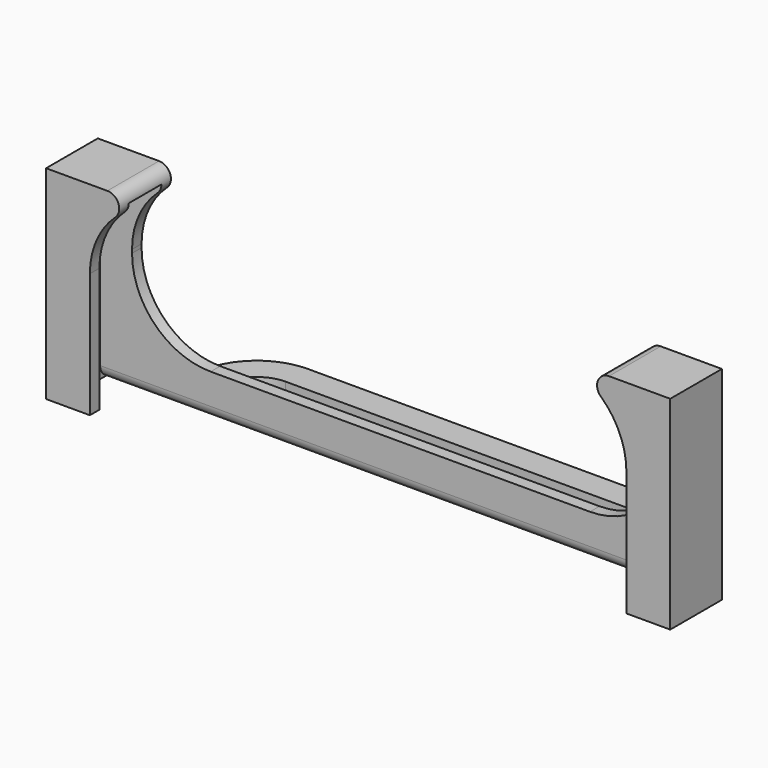
from build123d import *

# Parameters (mm, degrees)
F4_DEPTH     = 2.8
F5_W         = 146.8
F5_H         = 15.2
F5_W_2       = 141.2
F5_H_2       = 9.6
F6_DEPTH     = 47.8
F8_DEPTH     = 15.201
F9_DEPTH     = 2.8
F10_DEPTH    = 15.2
F11_T1_DEPTH = 141.2
F11_T3_DEPTH = 87.1722168618


# Not quite as in the source:
# - a fillet or chamfer that OpenCascade refuses, or shapes differently, is made with other operations: its cross-section is extruded or revolved along the edge and cut away or added
# - a feature names something its author has since deleted; it is built from what else it names


with BuildPart() as f4:
    # F3 (on Top) → F4 (new body)
    with BuildSketch(Plane.XY):
        with BuildLine():
            ThreePointArc((55, 5), (50.6066017178, 15.6066017178), (40, 20))
            Line((40, 20), (-40, 20))
            ThreePointArc((-40, 20), (-50.6066017178, 15.6066017178), (-55, 5))
            Line((-55, 5), (-55, 0))
            Line((-55, 0), (55, 0))
            Line((55, 0), (55, 5))
        make_face()
        with BuildLine():
            ThreePointArc((-48.3666002653, 6.5), (-45.4543560573, 11.5192024052), (-40, 13.5))
            Line((-40, 13.5), (40, 13.5))
            ThreePointArc((40, 13.5), (45.4543560573, 11.5192024052), (48.3666002653, 6.5))
            Line((48.3666002653, 6.5), (-48.3666002653, 6.5))
        make_face(mode=Mode.SUBTRACT)
    extrude(amount=F4_DEPTH)

    # F5 (on Top) → F6 (join)
    with BuildSketch(Plane.XY):
        with Locations((0, -7.6)):
            Rectangle(F5_W, F5_H)
        with Locations((0, -7.6)):
            Rectangle(F5_W_2, F5_H_2, mode=Mode.SUBTRACT)
    extrude(amount=F6_DEPTH)

    # F7 (on Front) → F8 (cut, through all)
    with BuildSketch(Plane.XZ):
        with BuildLine():
            Line((44.6, 47.8), (-44.6, 47.8))
            ThreePointArc((-44.6, 47.8), (-49.68920426, 47.0862306293), (-54.3857038582, 45))
            Line((-54.3857038582, 45), (54.3857038582, 45))
            ThreePointArc((54.3857038582, 45), (49.68920426, 47.0862306293), (44.6, 47.8))
        make_face()
        with BuildLine():
            ThreePointArc((-44.6, 10), (-57.681475452, 15.418524548), (-63.1, 28.5))
            Line((-63.1, 28.5), (-63.1, 10))
            Line((-63.1, 10), (-63.1, 0))
            Line((-63.1, 0), (63.1, 0))
            Line((63.1, 0), (63.1, 10))
            Line((63.1, 10), (63.1, 28.5))
            ThreePointArc((63.1, 28.5), (57.681475452, 15.418524548), (44.6, 10))
            Line((44.6, 10), (-44.6, 10))
        make_face()
        with BuildLine():
            Line((54.3857038582, 45), (-54.3857038582, 45))
            ThreePointArc((-54.3857038582, 45), (-60.7753751328, 38.2781534467), (-63.1, 29.3))
            Line((-63.1, 29.3), (-63.1, 28.5))
            ThreePointArc((-63.1, 28.5), (-57.681475452, 15.418524548), (-44.6, 10))
            Line((-44.6, 10), (44.6, 10))
            ThreePointArc((44.6, 10), (57.681475452, 15.418524548), (63.1, 28.5))
            Line((63.1, 28.5), (63.1, 29.3))
            ThreePointArc((63.1, 29.3), (60.7753751328, 38.2781534467), (54.3857038582, 45))
        make_face()
    extrude(amount=F8_DEPTH, mode=Mode.SUBTRACT)

    # F7 (on Front) → F9 (join)
    with BuildSketch(Plane.XZ):
        with BuildLine():
            ThreePointArc((-44.6, 10), (-57.681475452, 15.418524548), (-63.1, 28.5))
            Line((-63.1, 28.5), (-63.1, 10))
            Line((-63.1, 10), (-63.1, 0))
            Line((-63.1, 0), (63.1, 0))
            Line((63.1, 0), (63.1, 10))
            Line((63.1, 10), (63.1, 28.5))
            ThreePointArc((63.1, 28.5), (57.681475452, 15.418524548), (44.6, 10))
            Line((44.6, 10), (-44.6, 10))
        make_face()
    extrude(amount=F9_DEPTH)

    # F7 (on Front) → F10 (join)
    with BuildSketch(Plane.XZ):
        with BuildLine():
            ThreePointArc((-54.3857038582, 45), (-49.68920426, 47.0862306293), (-44.6, 47.8))
            Line((-44.6, 47.8), (-63.1, 47.8))
            Line((-63.1, 47.8), (-73.4, 47.8))
            Line((-73.4, 47.8), (-73.4, 45))
            Line((-73.4, 45), (-54.3857038582, 45))
        make_face()
        with BuildLine():
            Line((63.1, 47.8), (44.6, 47.8))
            ThreePointArc((44.6, 47.8), (49.68920426, 47.0862306293), (54.3857038582, 45))
            Line((54.3857038582, 45), (73.4, 45))
            Line((73.4, 45), (73.4, 47.8))
            Line((73.4, 47.8), (63.1, 47.8))
        make_face()
    extrude(amount=F10_DEPTH)

    # F11: fillet of radius 2.8 on 7 edges, made by hand

    # F11_s2 → F11_t1 (cut)
    with BuildSketch(Plane.YZ.offset(-70.6)):
        with BuildLine():
            ThreePointArc((-2.8, 2.8), (-1.9798989873, 0.8201010127), (0, 0))
            Line((0, 0), (-2.8, 0))
            Line((-2.8, 0), (-2.8, 2.8))
        make_face()
    extrude(amount=F11_T1_DEPTH, mode=Mode.SUBTRACT)

    # F11_s4 → F11_t3 (cut)
    with BuildSketch(Plane.XZ.offset(-35.9861084309)):
        with BuildLine():
            ThreePointArc((-58.9944433724, 47.8), (-56.3849626441, 46.0151897993), (-57.1022160746, 42.9361502347))
            ThreePointArc((-57.1022160746, 42.9361502347), (-51.3075040312, 46.5412119548), (-44.6, 47.8))
            Line((-44.6, 47.8), (-58.9944433724, 47.8))
        make_face()
        with BuildLine():
            ThreePointArc((57.1022160746, 42.9361502347), (56.3849626441, 46.0151897993), (58.9944433724, 47.8))
            Line((58.9944433724, 47.8), (44.6, 47.8))
            ThreePointArc((44.6, 47.8), (51.3075040312, 46.5412119548), (57.1022160746, 42.9361502347))
        make_face()
    extrude(amount=F11_T3_DEPTH, mode=Mode.SUBTRACT)


solid = f4.part
